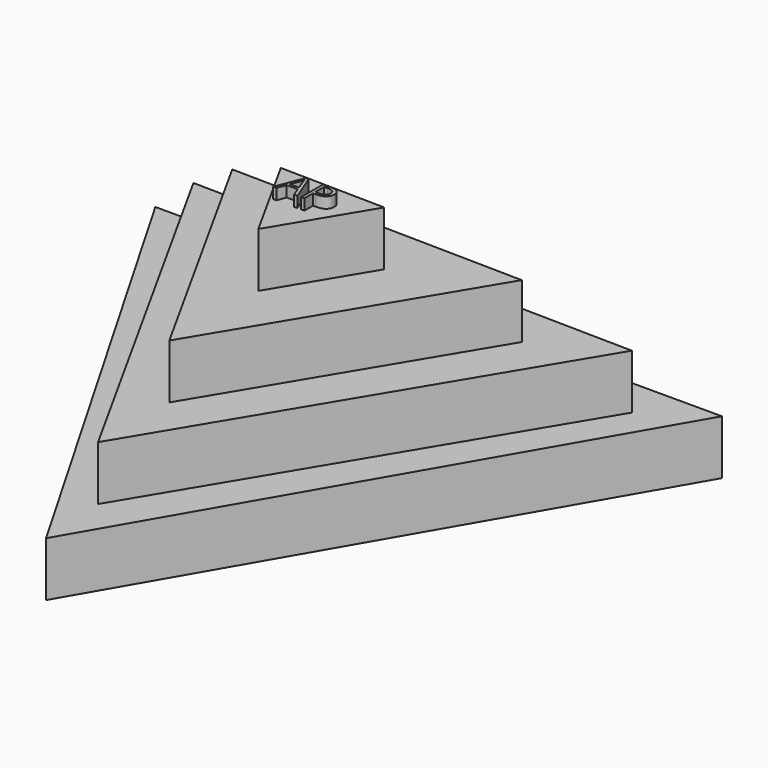
from build123d import *

# Parameters (mm, degrees)
F1_DEPTH     = 6.35
F3_DEPTH     = 6.35
F5_DEPTH     = 6.35
F7_DEPTH     = 6.35
F8_TEXT_SIZE = 4.4765998609
F9_DEPTH     = 7.62


# Not quite as in the source:
# - Text() gives the source's letters only with a copy of the font that has no kerning and outlines rounded to 1/6400 em; it was checked with that copy


with BuildPart() as f1:
    # F0 (on Top) → F1 (new body)
    with BuildSketch(Plane.XY):
        Polygon((33.0106055917, 19.0586820245), (-33.0106055917, 19.0586820245), (0, -38.117364049), align=None)
    extrude(amount=F1_DEPTH)

    # F2 (on face) → F3 (join)
    with BuildSketch(Plane.XY.offset(6.35)):
        Polygon((-0.5123303342, -29.9052900181), (26.1549060303, 14.5089539245), (-25.6425756961, 15.3963360935), align=None)
    extrude(amount=F3_DEPTH)

    # F4 (on face) → F5 (join)
    with BuildSketch(Plane.XY.offset(12.7)):
        Polygon((-0.3382971617, -19.7467806562), (17.2703622721, 9.5804163921), (-16.9320651104, 10.1663642641), align=None)
    extrude(amount=F5_DEPTH)

    # F6 (on face) → F7 (join)
    with BuildSketch(Plane.XY.offset(19.05)):
        Polygon((-0.1207556961, -7.0486439539), (6.1646825743, 3.4197444765), (-6.0439268783, 3.6288994774), align=None)
    extrude(amount=F7_DEPTH)

    # F8 (on face) → F9 (join)
    with BuildSketch(Plane.XY.offset(19.05)):
        with Locations((-2.7491576038, -1.6115759499)):
            Text('AP', F8_TEXT_SIZE, font='Open Sans', text_align=(TextAlign.LEFT, TextAlign.BOTTOM))
    extrude(amount=F9_DEPTH)


solid = f1.part
